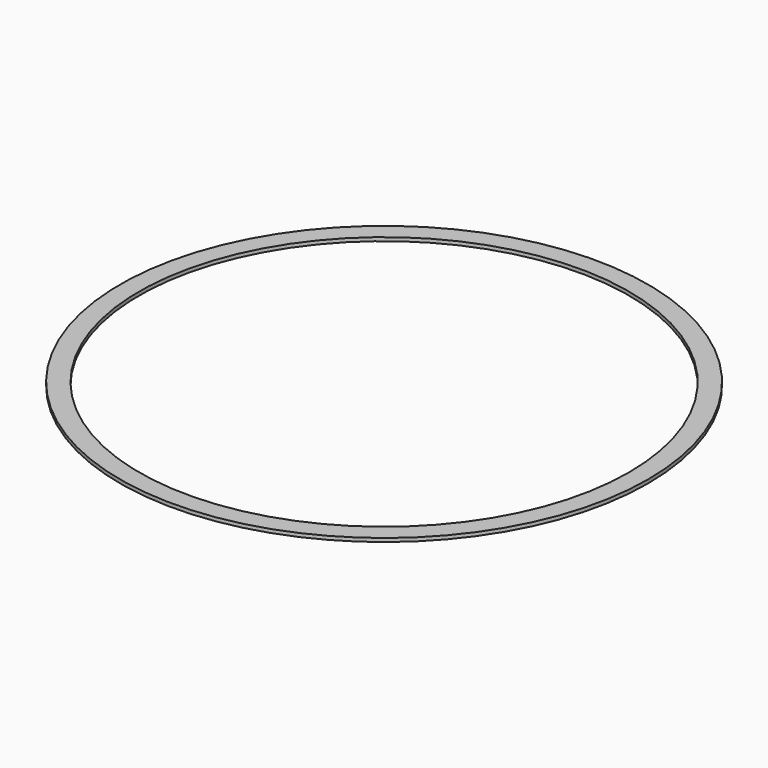
from build123d import *

# Parameters (mm, degrees)
F0_R     = 351.94748
F0_R_2   = 326.54748
F1_DEPTH = 4.7625


# Not quite as in the source:
# - a length typed as a fraction of an inch, garbled in the dataset ("3 / 203.2 mm" for 3/8 in), is restored


with BuildPart() as f1:
    # F0 (on Top) → F1 (new body)
    with BuildSketch(Plane.XY):
        Circle(F0_R)
        Circle(F0_R_2, mode=Mode.SUBTRACT)
    extrude(amount=F1_DEPTH)


solid = f1.part
